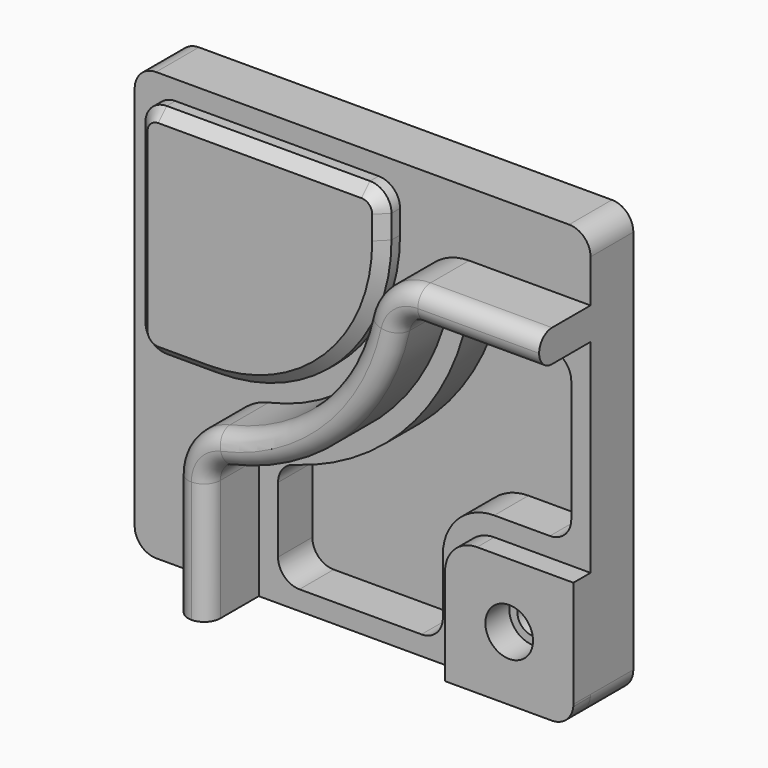
from build123d import *

# Parameters (mm, degrees)
F1_DEPTH        = 25
F2_DEPTH        = 10
F3_DEPTH        = 20
F4_DEPTH        = 30
F5_R            = 7.49999
F6_SIZE         = 5
F7_R            = 10
F8_DEPTH        = 10
F10_D           = 14.75
F10_CBORE_D     = 22.25
F10_CBORE_DEPTH = 14


# Not quite as in the source:
# - a fillet or chamfer is up to 0.001 mm smaller than in the source, because OpenCascade refuses the exact size


with BuildPart() as f1:
    # F0 (on Front) → F1 (new body)
    with BuildSketch(Plane.XZ):
        with BuildLine():
            Line((96.5, 100), (-96.5, 100))
            ThreePointArc((-96.5, 100), (-103.5710678119, 97.0710678119), (-106.5, 90))
            Line((-106.5, 90), (-106.5, -90))
            ThreePointArc((-106.5, -90), (-103.5710678119, -97.0710678119), (-96.5, -100))
            Line((-96.5, -100), (-63.5, -100))
            Line((-63.5, -100), (-63.5, -43.2740040786))
            ThreePointArc((-63.5, -43.2740040786), (-57.9897187751, -27.6167098657), (-43.8879310345, -18.8615031996))
            ThreePointArc((-43.8879310345, -18.8615031996), (0.846717088, 5.653282912), (25.3615031996, 50.3879310345))
            ThreePointArc((25.3615031996, 50.3879310345), (34.1167098657, 64.4897187751), (49.7740040786, 70))
            Line((49.7740040786, 70), (106.5, 70))
            Line((106.5, 70), (106.5, 90))
            ThreePointArc((106.5, 90), (103.5710678119, 97.0710678119), (96.5, 100))
        make_face()
        with BuildLine():
            ThreePointArc((17.5, 70), (-6.2243507239, 12.7243507239), (-63.5, -11))
            Line((-63.5, -11), (-87.5, -11))
            ThreePointArc((-87.5, -11), (-94.5710678119, -8.0710678119), (-97.5, -1))
            Line((-97.5, -1), (-97.5, 81))
            ThreePointArc((-97.5, 81), (-94.5710678119, 88.0710678119), (-87.5, 91))
            Line((-87.5, 91), (7.5, 91))
            ThreePointArc((7.5, 91), (14.5710678119, 88.0710678119), (17.5, 81))
            Line((17.5, 81), (17.5, 70))
        make_face(mode=Mode.SUBTRACT)
        with BuildLine():
            ThreePointArc((-96.5, -100), (-103.5710678119, -97.0710678119), (-106.5, -90))
            Line((-106.5, -90), (-106.5, -100))
            Line((-106.5, -100), (-96.5, -100))
        make_face()
        with BuildLine():
            Line((106.5, 55), (106.5, 70))
            Line((106.5, 70), (49.7740040786, 70))
            ThreePointArc((49.7740040786, 70), (34.1167098657, 64.4897187751), (25.3615031996, 50.3879310345))
            ThreePointArc((25.3615031996, 50.3879310345), (0.846717088, 5.653282912), (-43.8879310345, -18.8615031996))
            ThreePointArc((-43.8879310345, -18.8615031996), (-57.9897187751, -27.6167098657), (-63.5, -43.2740040786))
            Line((-63.5, -43.2740040786), (-63.5, -100))
            Line((-63.5, -100), (-48.5, -100))
            Line((-48.5, -100), (-48.5, -43.2740040786))
            ThreePointArc((-48.5, -43.2740040786), (-46.29588751, -37.0110863935), (-40.6551724138, -33.509003727))
            ThreePointArc((-40.6551724138, -33.509003727), (11.4533188058, -4.9533188058), (40.009003727, 47.1551724138))
            ThreePointArc((40.009003727, 47.1551724138), (43.5110863935, 52.79588751), (49.7740040786, 55))
            Line((49.7740040786, 55), (106.5, 55))
        make_face()
        with BuildLine():
            Line((106.5, -40), (106.5, 55))
            Line((106.5, 55), (49.7740040786, 55))
            ThreePointArc((49.7740040786, 55), (43.5110863935, 52.79588751), (40.009003727, 47.1551724138))
            ThreePointArc((40.009003727, 47.1551724138), (11.4533188058, -4.9533188058), (-40.6551724138, -33.509003727))
            ThreePointArc((-40.6551724138, -33.509003727), (-46.29588751, -37.0110863935), (-48.5, -43.2740040786))
            Line((-48.5, -43.2740040786), (-48.5, -100))
            Line((-48.5, -100), (46.5, -100))
            Line((46.5, -100), (46.5, -55))
            ThreePointArc((46.5, -55), (50.8933982822, -44.3933982822), (61.5, -40))
            Line((61.5, -40), (106.5, -40))
        make_face()
        with BuildLine():
            Line((56.7871564216, 46), (87.5, 46))
            ThreePointArc((87.5, 46), (94.5710678119, 43.0710678119), (97.5, 36))
            Line((97.5, 36), (97.5, -21))
            ThreePointArc((97.5, -21), (94.5710678119, -28.0710678119), (87.5, -31))
            Line((87.5, -31), (61.5, -31))
            ThreePointArc((61.5, -31), (44.5294372515, -38.0294372515), (37.5, -55))
            Line((37.5, -55), (37.5, -81))
            ThreePointArc((37.5, -81), (34.5710678119, -88.0710678119), (27.5, -91))
            Line((27.5, -91), (-29.5, -91))
            ThreePointArc((-29.5, -91), (-36.5710678119, -88.0710678119), (-39.5, -81))
            Line((-39.5, -81), (-39.5, -50.2871564216))
            ThreePointArc((-39.5, -50.2871564216), (-37.474960815, -44.25391517), (-32.22, -40.6641839079))
            ThreePointArc((-32.22, -40.6641839079), (17.8172798365, -11.3172798365), (47.1641839079, 38.72))
            ThreePointArc((47.1641839079, 38.72), (50.75391517, 43.974960815), (56.7871564216, 46))
        make_face(mode=Mode.SUBTRACT)
        with BuildLine():
            Line((106.5, -90), (106.5, -40))
            Line((106.5, -40), (61.5, -40))
            ThreePointArc((61.5, -40), (50.8933982822, -44.3933982822), (46.5, -55))
            Line((46.5, -55), (46.5, -100))
            Line((46.5, -100), (96.5, -100))
            ThreePointArc((96.5, -100), (97.0006277506, -99.9874607311), (97.5, -99.9498743711))
            ThreePointArc((97.5, -99.9498743711), (103.5710678119, -97.0710678119), (106.4498743711, -91))
            ThreePointArc((106.4498743711, -91), (106.4874607311, -90.5006277506), (106.5, -90))
        make_face()
        with BuildLine():
            Line((106.5, -91), (106.5, -90))
            ThreePointArc((106.5, -90), (106.4874607311, -90.5006277506), (106.4498743711, -91))
            Line((106.4498743711, -91), (106.5, -91))
        make_face()
        with BuildLine():
            Line((106.5, -91), (106.4498743711, -91))
            ThreePointArc((106.4498743711, -91), (103.5710678119, -97.0710678119), (97.5, -99.9498743711))
            Line((97.5, -99.9498743711), (97.5, -100))
            Line((97.5, -100), (106.5, -100))
            Line((106.5, -100), (106.5, -91))
        make_face()
        with BuildLine():
            ThreePointArc((97.5, -99.9498743711), (97.0006277506, -99.9874607311), (96.5, -100))
            Line((96.5, -100), (97.5, -100))
            Line((97.5, -100), (97.5, -99.9498743711))
        make_face()
        with BuildLine():
            Line((-87.5, -11), (-63.5, -11))
            ThreePointArc((-63.5, -11), (-6.2243507239, 12.7243507239), (17.5, 70))
            Line((17.5, 70), (17.5, 81))
            ThreePointArc((17.5, 81), (14.5710678119, 88.0710678119), (7.5, 91))
            Line((7.5, 91), (-87.5, 91))
            ThreePointArc((-87.5, 91), (-94.5710678119, 88.0710678119), (-97.5, 81))
            Line((-97.5, 81), (-97.5, -1))
            ThreePointArc((-97.5, -1), (-94.5710678119, -8.0710678119), (-87.5, -11))
        make_face()
        with BuildLine():
            ThreePointArc((97.5, 36), (94.5710678119, 43.0710678119), (87.5, 46))
            Line((87.5, 46), (56.7871564216, 46))
            ThreePointArc((56.7871564216, 46), (50.75391517, 43.974960815), (47.1641839079, 38.72))
            ThreePointArc((47.1641839079, 38.72), (17.8172798365, -11.3172798365), (-32.22, -40.6641839079))
            ThreePointArc((-32.22, -40.6641839079), (-37.474960815, -44.25391517), (-39.5, -50.2871564216))
            Line((-39.5, -50.2871564216), (-39.5, -81))
            ThreePointArc((-39.5, -81), (-36.5710678119, -88.0710678119), (-29.5, -91))
            Line((-29.5, -91), (27.5, -91))
            ThreePointArc((27.5, -91), (34.5710678119, -88.0710678119), (37.5, -81))
            Line((37.5, -81), (37.5, -55))
            ThreePointArc((37.5, -55), (44.5294372515, -38.0294372515), (61.5, -31))
            Line((61.5, -31), (87.5, -31))
            ThreePointArc((87.5, -31), (94.5710678119, -28.0710678119), (97.5, -21))
            Line((97.5, -21), (97.5, 36))
        make_face()
    extrude(amount=-F1_DEPTH)

    # F0 (on Front) → F2 (join)
    with BuildSketch(Plane.XZ):
        with BuildLine():
            Line((-87.5, -11), (-63.5, -11))
            ThreePointArc((-63.5, -11), (-6.2243507239, 12.7243507239), (17.5, 70))
            Line((17.5, 70), (17.5, 81))
            ThreePointArc((17.5, 81), (14.5710678119, 88.0710678119), (7.5, 91))
            Line((7.5, 91), (-87.5, 91))
            ThreePointArc((-87.5, 91), (-94.5710678119, 88.0710678119), (-97.5, 81))
            Line((-97.5, 81), (-97.5, -1))
            ThreePointArc((-97.5, -1), (-94.5710678119, -8.0710678119), (-87.5, -11))
        make_face()
    extrude(amount=F2_DEPTH)

    # F0 (on Front) → F3 (cut)
    with BuildSketch(Plane.XZ):
        with BuildLine():
            ThreePointArc((97.5, 36), (94.5710678119, 43.0710678119), (87.5, 46))
            Line((87.5, 46), (56.7871564216, 46))
            ThreePointArc((56.7871564216, 46), (50.75391517, 43.974960815), (47.1641839079, 38.72))
            ThreePointArc((47.1641839079, 38.72), (17.8172798365, -11.3172798365), (-32.22, -40.6641839079))
            ThreePointArc((-32.22, -40.6641839079), (-37.474960815, -44.25391517), (-39.5, -50.2871564216))
            Line((-39.5, -50.2871564216), (-39.5, -81))
            ThreePointArc((-39.5, -81), (-36.5710678119, -88.0710678119), (-29.5, -91))
            Line((-29.5, -91), (27.5, -91))
            ThreePointArc((27.5, -91), (34.5710678119, -88.0710678119), (37.5, -81))
            Line((37.5, -81), (37.5, -55))
            ThreePointArc((37.5, -55), (44.5294372515, -38.0294372515), (61.5, -31))
            Line((61.5, -31), (87.5, -31))
            ThreePointArc((87.5, -31), (94.5710678119, -28.0710678119), (97.5, -21))
            Line((97.5, -21), (97.5, 36))
        make_face()
    extrude(amount=-F3_DEPTH, mode=Mode.SUBTRACT)

    # F0 (on Front) → F4 (join)
    with BuildSketch(Plane.XZ):
        with BuildLine():
            Line((106.5, 55), (106.5, 70))
            Line((106.5, 70), (49.7740040786, 70))
            ThreePointArc((49.7740040786, 70), (34.1167098657, 64.4897187751), (25.3615031996, 50.3879310345))
            ThreePointArc((25.3615031996, 50.3879310345), (0.846717088, 5.653282912), (-43.8879310345, -18.8615031996))
            ThreePointArc((-43.8879310345, -18.8615031996), (-57.9897187751, -27.6167098657), (-63.5, -43.2740040786))
            Line((-63.5, -43.2740040786), (-63.5, -100))
            Line((-63.5, -100), (-48.5, -100))
            Line((-48.5, -100), (-48.5, -43.2740040786))
            ThreePointArc((-48.5, -43.2740040786), (-46.29588751, -37.0110863935), (-40.6551724138, -33.509003727))
            ThreePointArc((-40.6551724138, -33.509003727), (11.4533188058, -4.9533188058), (40.009003727, 47.1551724138))
            ThreePointArc((40.009003727, 47.1551724138), (43.5110863935, 52.79588751), (49.7740040786, 55))
            Line((49.7740040786, 55), (106.5, 55))
        make_face()
    extrude(amount=F4_DEPTH)

    # F5 (radius 7.5 in the source; OpenCascade refuses exactly that, so slightly less here)
    f5_edges = [f1.edges().sort_by_distance(p)[0] for p in [
        (-63.5, -30, -71.637002),
        (-48.5, -30, -71.637002),
    ]]
    fillet(f5_edges, radius=F5_R)

    # F6
    f6_edges = [f1.edges().sort_by_distance(p)[0] for p in [
        (-97.5, -10, 40),
    ]]
    chamfer(f6_edges, length=F6_SIZE)

    # F7
    f7_edges = [f1.edges().sort_by_distance(p)[0] for p in [
        (-106.5, 12.5, -100),
        (106.5, 12.5, -100),
    ]]
    fillet(f7_edges, radius=F7_R)

    # F0 (on Front) → F8 (join)
    with BuildSketch(Plane.XZ):
        with BuildLine():
            Line((106.5, -90), (106.5, -40))
            Line((106.5, -40), (61.5, -40))
            ThreePointArc((61.5, -40), (50.8933982822, -44.3933982822), (46.5, -55))
            Line((46.5, -55), (46.5, -100))
            Line((46.5, -100), (96.5, -100))
            ThreePointArc((96.5, -100), (97.0006277506, -99.9874607311), (97.5, -99.9498743711))
            ThreePointArc((97.5, -99.9498743711), (103.5710678119, -97.0710678119), (106.4498743711, -91))
            ThreePointArc((106.4498743711, -91), (106.4874607311, -90.5006277506), (106.5, -90))
        make_face()
    extrude(amount=F8_DEPTH)

    # F10 (through all)
    with Locations(Plane.XZ.offset(10)):
        with Locations((76.5, -70)):
            CounterBoreHole(F10_D / 2, F10_CBORE_D / 2, F10_CBORE_DEPTH)


solid = f1.part
